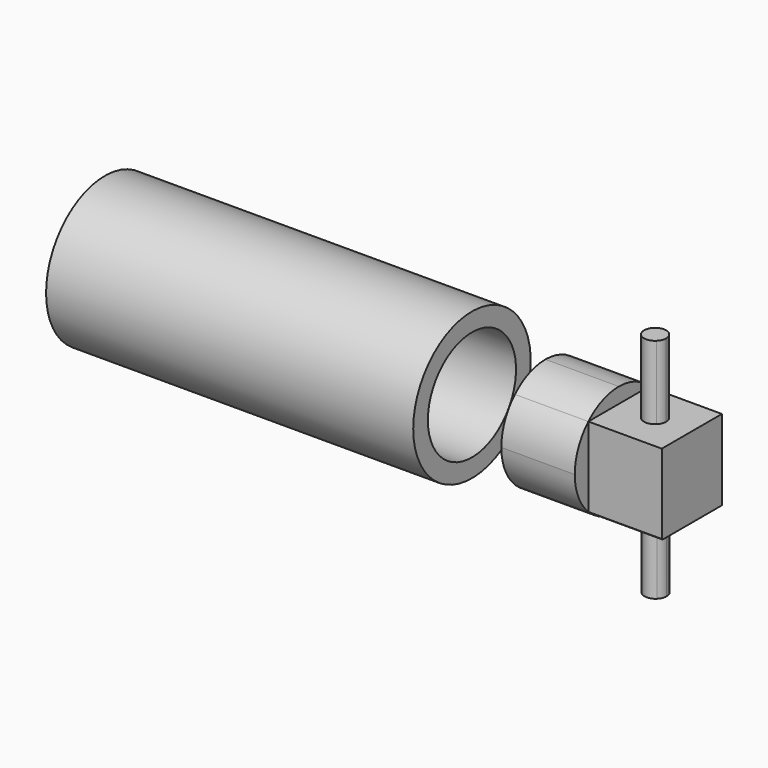
from build123d import *

# Parameters (mm, degrees)
F0_W     = 12.8274819265
F0_H     = 14.0839698744
F0_H_2   = 13.7507947324
F0_W_2   = 13.1840109309
F1_DEPTH = 25.4
F2_DEPTH = 25.4
F5_DEPTH = 25.4
F6_DEPTH = 25.4
F8_R     = 25.4
F9_DEPTH = 127
F11_D    = 38.1


with BuildPart() as f1:
    # F0 (on Right) → F1 (new body)
    with BuildSketch(Plane.YZ):
        with Locations((6.4137409633, -7.0419849372)):
            Rectangle(F0_W, F0_H)
        with Locations((6.4137409633, 6.8753973662)):
            Rectangle(F0_W, F0_H_2)
        with Locations((-6.5920054655, 6.8753973662)):
            Rectangle(F0_W_2, F0_H_2)
        with BuildLine():
            Line((-12.8274819265, -14.0839698744), (0, -14.0839698744))
            Line((0, -14.0839698744), (0, 0))
            Line((0, 0), (-13.1840109309, 0))
            Line((-13.1840109309, 0), (-13.1840109309, -13.7507947324))
            ThreePointArc((-13.1840109309, -13.7507947324), (-13.0068132756, -13.9185239308), (-12.8274819265, -14.0839698744))
        make_face()
    extrude(amount=F1_DEPTH)

    # F0 (on Right) → F2 (join)
    with BuildSketch(Plane.YZ):
        with BuildLine():
            Line((12.8274819265, 0), (19.05, 0))
            ThreePointArc((19.05, 0), (13.4703841816, 13.4703841816), (0, 19.05))
            Line((0, 19.05), (0, 13.7507947324))
            Line((0, 13.7507947324), (12.8274819265, 13.7507947324))
            Line((12.8274819265, 13.7507947324), (12.8274819265, 0))
        make_face()
        with BuildLine():
            ThreePointArc((12.8274819265, -14.0839698744), (17.4250685895, -7.6986677191), (19.05, 0))
            Line((19.05, 0), (12.8274819265, 0))
            Line((12.8274819265, 0), (12.8274819265, -14.0839698744))
        make_face()
        with BuildLine():
            Line((0, 13.7507947324), (0, 19.05))
            ThreePointArc((0, 19.05), (-7.104571076, 17.6756207763), (-13.1840109309, 13.7507947324))
            Line((-13.1840109309, 13.7507947324), (0, 13.7507947324))
        make_face()
        with BuildLine():
            ThreePointArc((0, -19.05), (6.877604012, -17.7651643126), (12.8274819265, -14.0839698744))
            Line((12.8274819265, -14.0839698744), (0, -14.0839698744))
            Line((0, -14.0839698744), (0, -19.05))
        make_face()
        with Locations((6.4137409633, -7.0419849372)):
            Rectangle(F0_W, F0_H)
        with Locations((6.4137409633, 6.8753973662)):
            Rectangle(F0_W, F0_H_2)
        with BuildLine():
            Line((-13.1840109309, 0), (-13.1840109309, 13.7507947324))
            ThreePointArc((-13.1840109309, 13.7507947324), (-17.5222416978, 7.4748609273), (-19.05, 0))
            Line((-19.05, 0), (-13.1840109309, 0))
        make_face()
        with Locations((-6.5920054655, 6.8753973662)):
            Rectangle(F0_W_2, F0_H_2)
        with BuildLine():
            ThreePointArc((-12.8274819265, -14.0839698744), (-6.877604012, -17.7651643126), (0, -19.05))
            Line((0, -19.05), (0, -14.0839698744))
            Line((0, -14.0839698744), (-12.8274819265, -14.0839698744))
        make_face()
        with BuildLine():
            Line((-12.8274819265, -14.0839698744), (0, -14.0839698744))
            Line((0, -14.0839698744), (0, 0))
            Line((0, 0), (-13.1840109309, 0))
            Line((-13.1840109309, 0), (-13.1840109309, -13.7507947324))
            ThreePointArc((-13.1840109309, -13.7507947324), (-13.0068132756, -13.9185239308), (-12.8274819265, -14.0839698744))
        make_face()
        with BuildLine():
            Line((-13.1840109309, 0), (-19.05, 0))
            ThreePointArc((-19.05, 0), (-17.5222416978, -7.4748609273), (-13.1840109309, -13.7507947324))
            Line((-13.1840109309, -13.7507947324), (-13.1840109309, 0))
        make_face()
    extrude(amount=-F2_DEPTH)

    # F3 (on face) → F5 (join)
    with BuildSketch(Plane.XY.offset(13.7507947324)):
        with BuildLine():
            ThreePointArc((15.3618449693, 2.5476631123), (12.7, 3.6317354978), (10.0381550307, 2.5476631123))
            Line((10.0381550307, 2.5476631123), (12.7, -0.1782645022))
            Line((12.7, -0.1782645022), (15.3618449693, 2.5476631123))
        make_face()
        with BuildLine():
            Line((12.7, -0.1782645022), (10.0381550307, 2.5476631123))
            ThreePointArc((10.0381550307, 2.5476631123), (8.89, -0.1782645022), (10.0381550307, -2.9041921166))
            Line((10.0381550307, -2.9041921166), (12.7, -0.1782645022))
        make_face()
        with BuildLine():
            Line((15.3618449693, -2.9041921166), (12.7, -0.1782645022))
            Line((12.7, -0.1782645022), (10.0381550307, -2.9041921166))
            ThreePointArc((10.0381550307, -2.9041921166), (12.7, -3.9882645022), (15.3618449693, -2.9041921166))
        make_face()
        with BuildLine():
            Line((15.3618449693, 2.5476631123), (12.7, -0.1782645022))
            Line((12.7, -0.1782645022), (15.3618449693, -2.9041921166))
            ThreePointArc((15.3618449693, -2.9041921166), (16.211248306, -1.6571949716), (16.51, -0.1782645022))
            ThreePointArc((16.51, -0.1782645022), (16.211248306, 1.3006659673), (15.3618449693, 2.5476631123))
        make_face()
    extrude(amount=F5_DEPTH)

    # F4 (on face) → F6 (join)
    with BuildSketch(Plane(origin=(0, 0, -14.0839698744), x_dir=(1, 0, 0), z_dir=(0, 0, -1))):
        with BuildLine():
            ThreePointArc((10.0194105643, -2.7074970503), (12.7, -3.81), (15.3805894357, -2.7074970503))
            Line((15.3805894357, -2.7074970503), (12.7, 0))
            Line((12.7, 0), (10.0194105643, -2.7074970503))
        make_face()
        with BuildLine():
            Line((12.7, 0), (15.3805894357, -2.7074970503))
            ThreePointArc((15.3805894357, -2.7074970503), (16.2163294605, -1.4668084827), (16.51, 0))
            ThreePointArc((16.51, 0), (16.2163294605, 1.4668084827), (15.3805894357, 2.7074970503))
            Line((15.3805894357, 2.7074970503), (12.7, 0))
        make_face()
        with BuildLine():
            Line((10.0194105643, 2.7074970503), (12.7, 0))
            Line((12.7, 0), (15.3805894357, 2.7074970503))
            ThreePointArc((15.3805894357, 2.7074970503), (12.7, 3.81), (10.0194105643, 2.7074970503))
        make_face()
        with BuildLine():
            Line((10.0194105643, -2.7074970503), (12.7, 0))
            Line((12.7, 0), (10.0194105643, 2.7074970503))
            ThreePointArc((10.0194105643, 2.7074970503), (8.89, 0), (10.0194105643, -2.7074970503))
        make_face()
    extrude(amount=F6_DEPTH)


with BuildPart() as f9:
    # F8 (on offset) → F9 (new body)
    with BuildSketch(Plane(origin=(-50.8, 0, 0), x_dir=(0, -1, 0), z_dir=(-1, 0, 0))):
        Circle(F8_R)
    extrude(amount=F9_DEPTH)

    # F11 (through all)
    with Locations(Plane.YZ.offset(-50.8)):
        with Locations((0, 0)):
            Hole(F11_D / 2)


solid = Compound([f1.part, f9.part])
